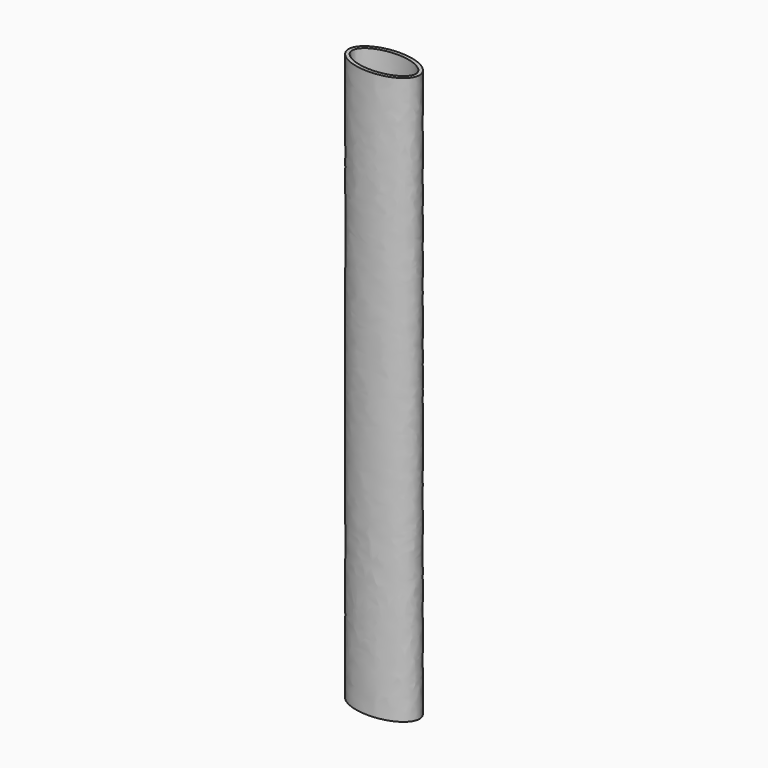
from build123d import *

# Parameters (mm, degrees)
F1_DEPTH = 203.2


# Not quite as in the source:
# - the dataset's text gives a spline's control points without its knots; the knots are read off the source's solid


with BuildPart() as f1:
    # F0 (on Top) → F1 (new body)
    with BuildSketch(Plane.XY):
        with BuildLine():
            add(Edge.make_bspline(
                [(-12.7, 0), (-12.7, -12.4877463863), (6.35, -6.2438731931), (25.4, 0), (6.35, 6.2438731931), (-12.7, 12.4877463863), (-12.7, 0)],
                knots=[0, 0, 0, 2.0943951024, 2.0943951024, 4.1887902048, 4.1887902048, 6.2831853072, 6.2831853072, 6.2831853072], degree=2, weights=[1, 0.5, 1, 0.5, 1, 0.5, 1]))
        make_face()
        with BuildLine():
            add(Edge.make_bspline(
                [(-11.43, 0), (-11.43, -0.3265636952), (-11.3192046794, -0.9796910856), (-10.8702000072, -1.8350174923), (-10.2949451779, -2.5282170965), (-9.5722052943, -3.21395612), (-8.4138776203, -4.0176381865), (-6.9524425656, -4.7014190668), (-5.6258616491, -5.1531060902), (-4.2234407931, -5.5293823785), (-2.7286196199, -5.7869294513), (-1.1805059108, -5.9176995392), (0, -5.9508558369), (1.1805059108, -5.9176995392), (2.7286196199, -5.7869294513), (4.2234407931, -5.5293823785), (5.6258616491, -5.1531060902), (6.9524425656, -4.7014190668), (8.4138776203, -4.0176381865), (9.5722052943, -3.21395612), (10.2949451779, -2.5282170965), (10.8702000072, -1.8350174923), (11.3192046794, -0.9796910856), (11.4853976603, 0), (11.3192046794, 0.9796910856), (10.8702000072, 1.8350174923), (10.2949451779, 2.5282170965), (9.5722052943, 3.21395612), (8.4138776203, 4.0176381865), (6.9524425656, 4.7014190668), (5.6258616491, 5.1531060902), (4.2234407931, 5.5293823785), (2.7286196199, 5.7869294513), (1.1805059108, 5.9176995392), (0, 5.9508558369), (-1.1805059108, 5.9176995392), (-2.7286196199, 5.7869294513), (-4.2234407931, 5.5293823785), (-5.6258616491, 5.1531060902), (-6.9524425656, 4.7014190668), (-8.4138776203, 4.0176381865), (-9.5722052943, 3.21395612), (-10.2949451779, 2.5282170965), (-10.8702000072, 1.8350174923), (-11.3192046794, 0.9796910856), (-11.43, 0.3265636952), (-11.43, 0)],
                knots=[0, 0, 0, 0, 0.03125, 0.0625, 0.078125, 0.09375, 0.125, 0.15625, 0.171875, 0.1875, 0.21875, 0.234375, 0.25, 0.265625, 0.28125, 0.3125, 0.328125, 0.34375, 0.375, 0.40625, 0.421875, 0.4375, 0.46875, 0.5, 0.53125, 0.5625, 0.578125, 0.59375, 0.625, 0.65625, 0.671875, 0.6875, 0.71875, 0.734375, 0.75, 0.765625, 0.78125, 0.8125, 0.828125, 0.84375, 0.875, 0.90625, 0.921875, 0.9375, 0.96875, 1, 1, 1, 1], degree=3))
        make_face(mode=Mode.SUBTRACT)
    extrude(amount=F1_DEPTH)


solid = f1.part
